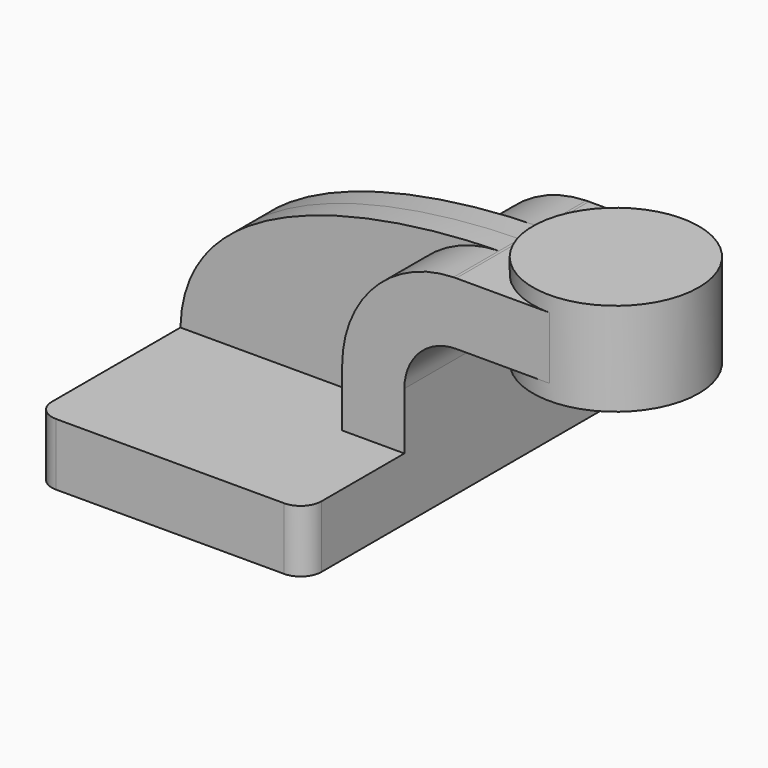
from build123d import *

# Parameters (mm, degrees)
F1_DEPTH = 63.5
F0_W     = 25.4
F0_H     = 19.05
F2_DEPTH = 25.4
F3_DEPTH = 7.9375
F5_R     = 6.35


# Not quite as in the source:
# - a feature names something its author has since deleted; it is built from what else it names


with BuildPart() as f1:
    # F0 (on Front) → F1 (new body, symmetric)
    with BuildSketch(Plane.XZ):
        Polygon((-41.275, -9.525), (41.275, -9.525), (41.275, 9.525), (22.225, 9.525), (-41.275, 9.525), align=None)
    extrude(amount=F1_DEPTH, both=True)

    # F0 (on Front) → F2 (join, symmetric)
    with BuildSketch(Plane.XZ):
        with BuildLine():
            Line((22.225, 9.525), (41.275, 9.525))
            Line((41.275, 9.525), (41.275, 27.0002))
            ThreePointArc((41.275, 27.0002), (45.9246798487, 38.2255201513), (57.15, 42.8752))
            Line((57.15, 42.8752), (60.325, 42.8752))
            Line((60.325, 42.8752), (60.325, 61.9252))
            Line((60.325, 61.9252), (57.15, 61.9252))
            add(Edge.make_bspline(
                [(56.3025201656, 61.914916137), (56.5862693172, 61.9189290335), (56.8687741652, 61.9223540897), (57.15, 61.9252)],
                knots=[110.666674481, 110.666674481, 110.666674481, 110.666674481, 111.5045361635, 111.5045361635, 111.5045361635, 111.5045361635], degree=3))
            ThreePointArc((56.3025201656, 61.914916137), (32.156462253, 51.3944348905), (22.225, 27.0002))
            Line((22.225, 27.0002), (22.225, 9.525))
        make_face()
        with Locations((73.025, 52.4002)):
            Rectangle(F0_W, F0_H)
    extrude(amount=F2_DEPTH, both=True)

    # F0 (on Front) → F3 (join, symmetric)
    with BuildSketch(Plane.XZ):
        with BuildLine():
            add(Edge.make_bspline(
                [(-41.275, 9.525), (-40.3617250948, 50.5995517259), (18.8242875965, 61.3848836588), (56.3025201656, 61.914916137)],
                knots=[0, 0, 0, 0, 110.666674481, 110.666674481, 110.666674481, 110.666674481], degree=3))
            Line((-41.275, 9.525), (22.225, 9.525))
            Line((22.225, 9.525), (22.225, 27.0002))
            ThreePointArc((22.225, 27.0002), (32.156462253, 51.3944348905), (56.3025201656, 61.914916137))
        make_face()
    extrude(amount=F3_DEPTH, both=True)

    # F0 (on Front) → F4 (revolve)
    with BuildSketch(Plane.XZ):
        Polygon((85.725, 61.9252), (85.725, 42.8752), (85.725, 38.1), (111.125, 38.1), (111.125, 66.675), (85.725, 66.675), align=None)
    revolve(axis=Axis((85.725, 0, 52.3875), (0, 0, -1)))

    # F5
    f5_edges = [f1.edges().sort_by_distance(p)[0] for p in [
        (-41.275, -63.5, 0),
        (41.275, -63.5, 0),
        (41.275, 63.5, 0),
        (-41.275, 63.5, 0),
    ]]
    fillet(f5_edges, radius=F5_R)


solid = f1.part
